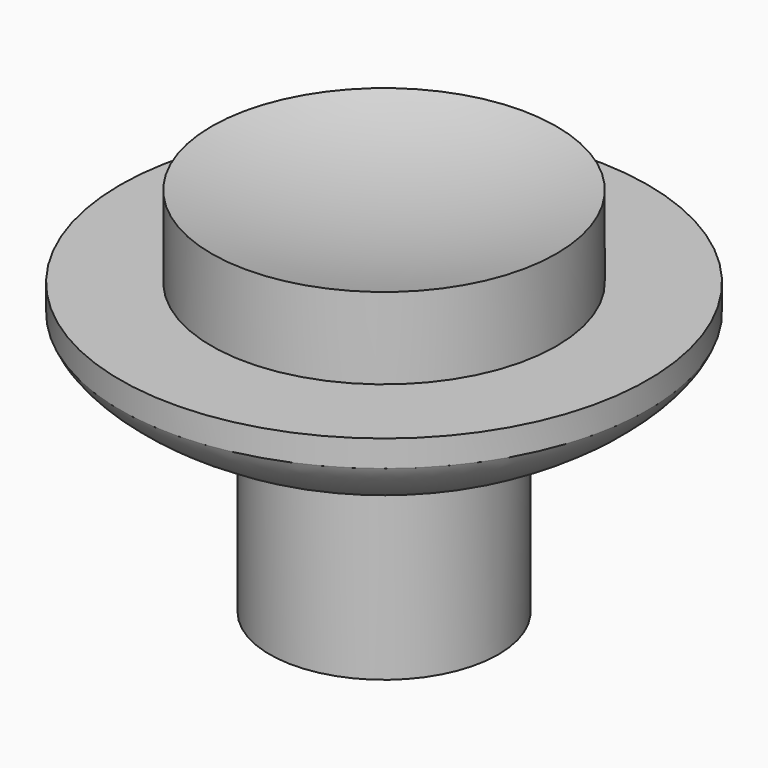
from build123d import *

# Parameters (mm, degrees)
F3_R          = 9.8
F4_DEPTH      = 10
F4_DEPTH_BACK = 0.3
F6_R          = 15
F6_R_2        = 9.8
F7_DEPTH      = 1.5
F9_ANGLE      = 180
F10_R         = 6.5
F11_DEPTH     = 15


# Not quite as in the source:
# - a feature names something its author has since deleted; it is built from what else it names


with BuildPart() as f1:
    # F0 (on Top) → F1 (revolve)
    with BuildSketch(Plane.XY):
        with BuildLine():
            Line((0, 37), (0, -37))
            ThreePointArc((0, -37), (37, 0), (0, 37))
        make_face()
    revolve(axis=Axis((0, 0, 0), (0, -1, 0)))


with BuildPart() as f4:
    # F3 (on offset) → F4 (new body, two sides)
    with BuildSketch(Plane.XY.offset(40)) as f4_sk:
        Circle(F3_R)
    extrude(amount=-F4_DEPTH)
    extrude(f4_sk.sketch, amount=F4_DEPTH_BACK)

    # F5: cut F1
    add(f1.part, mode=Mode.SUBTRACT)

    # F6 (on face) → F7 (join)
    with BuildSketch(Plane.XY.offset(40.3)):
        Circle(F6_R)
        Circle(F6_R_2, mode=Mode.SUBTRACT)
        Circle(F6_R_2)
    extrude(amount=F7_DEPTH)


with BuildPart() as f4_1:
    # F9: moved
    add(f4.part.rotate(Axis((0, 0, 41.8), (0, 1, 0)), F9_ANGLE))

    # F10 (on face) → F11 (join)
    with BuildSketch(Plane(origin=(0, 0, 41.8), x_dir=(1, 0, 0), z_dir=(0, 0, -1))):
        Circle(F10_R)
    extrude(amount=F11_DEPTH)

    # F12 (on Front) → F14 (revolve)
    with BuildSketch(Plane.XZ):
        with BuildLine():
            Line((-6.5, 36.8), (-6.5, 41.8))
            Line((-6.5, 41.8), (-15, 41.8))
            add(Edge.make_bspline(
                [(-15, 41.8), (-14.5252337679, 40.5401661992), (-10.4554320312, 37.7730797784), (-8.2265594974, 37.2042804956), (-6.5, 36.8)],
                knots=[0, 0, 0, 0, 0.5265068143, 1, 1, 1, 1], degree=3))
        make_face()
    revolve(axis=Axis((0, 0, 37.5033216551), (0, 0, 1)))


solid = f4_1.part
